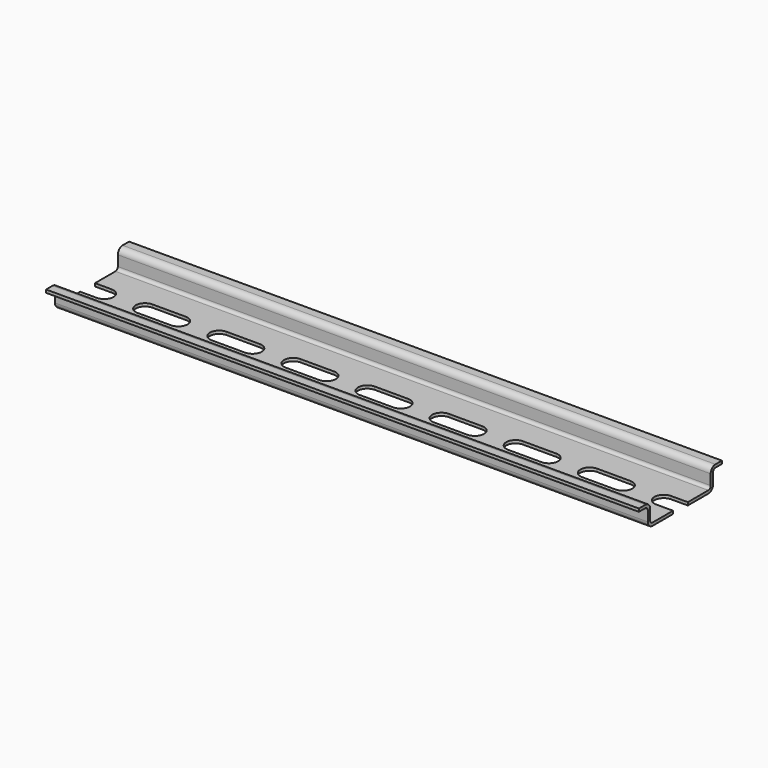
from build123d import *

# Parameters (mm, degrees)
F1_DEPTH = 101.6
F3_DEPTH = 1.0162968718


# Not quite as in the source:
# - ends of sketch curves that miss each other by under 0.0002 mm in the source are joined


with BuildPart() as f1:
    # F0 (on Right) → F1 (new body, symmetric)
    with BuildSketch(Plane.YZ):
        with BuildLine():
            Line((-13.9794936462, -2.032), (-13.9794936462, -5.5877193844))
            ThreePointArc((-13.9794936462, -5.5877193844), (-13.384185281, -7.0242872241), (-11.9474936901, -7.6192968718))
            Line((-11.9474936901, -7.6192968718), (11.9474936901, -7.6192968718))
            ThreePointArc((11.9474936901, -7.6192968718), (13.3841865534, -7.024285952), (13.9794936469, -5.5877157858))
            Line((13.9794936469, -5.5877157858), (13.9794936469, -2.0319964014))
            ThreePointArc((13.9794936469, -2.0319964014), (14.2772790988, -1.313078725), (14.9961967752, -1.0152932732))
            Line((14.9961967752, -1.0152932732), (17.7780878922, -1.0152932732))
            Line((17.7780878922, -1.0152932732), (17.7780878922, 0))
            Line((17.7780878922, 0), (14.9923725588, 0))
            ThreePointArc((14.9923725588, 0), (13.5581523434, -0.5963598833), (12.9641968184, -2.0315774874))
            Line((12.9641968184, -2.0315774874), (12.9641968184, -5.5872968718))
            ThreePointArc((12.9641968184, -5.5872968718), (12.6664113666, -6.3062145482), (11.9474936901, -6.604))
            Line((11.9474936901, -6.604), (-11.9474936901, -6.604))
            ThreePointArc((-11.9474936901, -6.604), (-12.6664113666, -6.3062145482), (-12.9641968184, -5.5872968718))
            Line((-12.9641968184, -5.5872968718), (-12.9641968184, -2.0315774874))
            ThreePointArc((-12.9641968184, -2.0315774874), (-13.5595051836, -0.5950096476), (-14.9961967744, 0))
            Line((-14.9961967744, 0), (-17.7819121078, 0))
            Line((-17.7819121078, 0), (-17.7819121078, -1.0152932732))
            Line((-17.7819121078, -1.0152932732), (-14.9961967744, -1.0152932732))
            ThreePointArc((-14.9961967744, -1.0152932732), (-14.277279098, -1.3130823236), (-13.9794936462, -2.032))
        make_face()
    extrude(amount=F1_DEPTH, both=True)

    # F2 (on face) → F3 (cut, through all)
    with BuildSketch(Plane.XY.offset(-6.604)):
        with BuildLine():
            Line((-5.715, -3.175), (5.715, -3.175))
            ThreePointArc((5.715, -3.175), (8.89, 0), (5.715, 3.175))
            Line((5.715, 3.175), (-5.715, 3.175))
            ThreePointArc((-5.715, 3.175), (-8.89, 0), (-5.715, -3.175))
        make_face()
        with BuildLine():
            Line((19.685, -3.175), (31.115, -3.175))
            ThreePointArc((31.115, -3.175), (34.29, 0), (31.115, 3.175))
            Line((31.115, 3.175), (19.685, 3.175))
            ThreePointArc((19.685, 3.175), (16.51, 0), (19.685, -3.175))
        make_face()
        with BuildLine():
            Line((45.085, -3.175), (56.515, -3.175))
            ThreePointArc((56.515, -3.175), (59.69, 0), (56.515, 3.175))
            Line((56.515, 3.175), (45.085, 3.175))
            ThreePointArc((45.085, 3.175), (41.91, 0), (45.085, -3.175))
        make_face()
        with BuildLine():
            Line((70.485, -3.175), (81.915, -3.175))
            ThreePointArc((81.915, -3.175), (85.09, 0), (81.915, 3.175))
            Line((81.915, 3.175), (70.485, 3.175))
            ThreePointArc((70.485, 3.175), (67.31, 0), (70.485, -3.175))
        make_face()
        with BuildLine():
            Line((95.885, -3.175), (107.315, -3.175))
            ThreePointArc((107.315, -3.175), (110.49, 0), (107.315, 3.175))
            Line((107.315, 3.175), (95.885, 3.175))
            ThreePointArc((95.885, 3.175), (92.71, 0), (95.885, -3.175))
        make_face()
        with BuildLine():
            Line((-19.685, 3.175), (-31.115, 3.175))
            ThreePointArc((-31.115, 3.175), (-34.29, 0), (-31.115, -3.175))
            Line((-31.115, -3.175), (-19.685, -3.175))
            ThreePointArc((-19.685, -3.175), (-16.51, 0), (-19.685, 3.175))
        make_face()
        with BuildLine():
            Line((-45.085, 3.175), (-56.515, 3.175))
            ThreePointArc((-56.515, 3.175), (-59.69, 0), (-56.515, -3.175))
            Line((-56.515, -3.175), (-45.085, -3.175))
            ThreePointArc((-45.085, -3.175), (-41.91, 0), (-45.085, 3.175))
        make_face()
        with BuildLine():
            Line((-70.485, 3.175), (-81.915, 3.175))
            ThreePointArc((-81.915, 3.175), (-85.09, 0), (-81.915, -3.175))
            Line((-81.915, -3.175), (-70.485, -3.175))
            ThreePointArc((-70.485, -3.175), (-67.31, 0), (-70.485, 3.175))
        make_face()
        with BuildLine():
            Line((-95.885, 3.175), (-107.315, 3.175))
            ThreePointArc((-107.315, 3.175), (-110.49, 0), (-107.315, -3.175))
            Line((-107.315, -3.175), (-95.885, -3.175))
            ThreePointArc((-95.885, -3.175), (-92.71, 0), (-95.885, 3.175))
        make_face()
    extrude(amount=-F3_DEPTH, mode=Mode.SUBTRACT)


solid = f1.part
